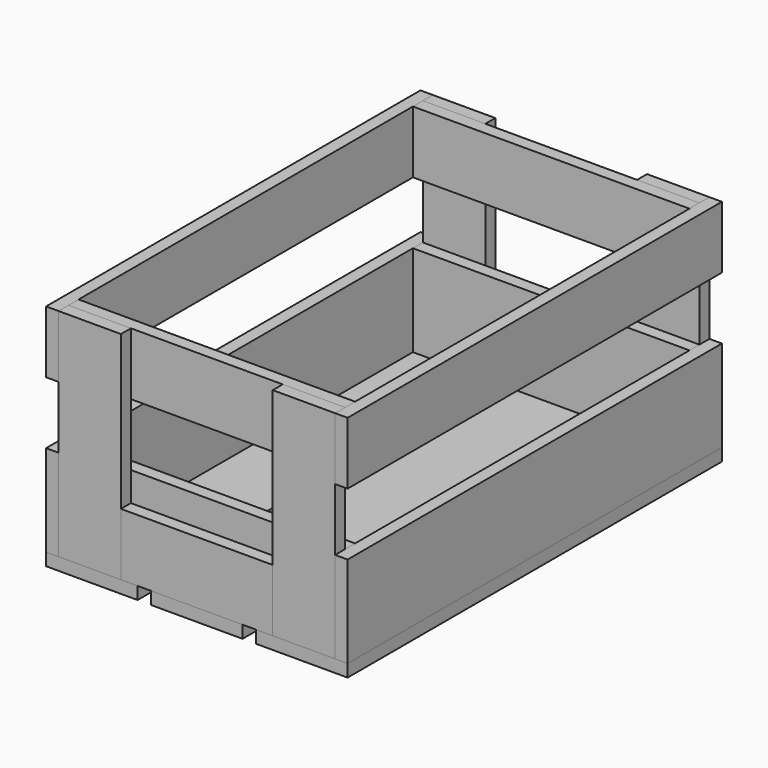
from build123d import *

# Parameters (mm, degrees)
F0_W      = 290
F0_H      = 225
F1_DEPTH  = 220
F2_W      = 12
F2_H      = 60
F3_DEPTH  = 450
F2_H_2    = 12
F2_W_2    = 88
F2_H_3    = 88
F4_DEPTH  = 450
F5_W      = 60
F5_H      = 12
F6_DEPTH  = 208
F5_W_2    = 73
F7_DEPTH  = 60
F8_START  = -120
F8_DEPTH  = 88
F9_DEPTH  = 12
F10_DEPTH = 25


with BuildPart() as f1:
    # F0 (on Top) → F1 (new body)
    with BuildSketch(Plane.XY):
        with Locations((145, 112.5)):
            Rectangle(F0_W, F0_H)
        with Locations((145, 337.5)):
            Rectangle(F0_W, F0_H)
    extrude(amount=F1_DEPTH)


with BuildPart() as f3:
    # F2 (on face) → F3 (new body, through all)
    with BuildSketch(Plane(origin=(0, 450, 0), x_dir=(-1, 0, 0), z_dir=(0, 1, 0))):
        with Locations((-284, 190)):
            Rectangle(F2_W, F2_H)
    extrude(amount=-F3_DEPTH)


with BuildPart() as f3b:
    # F2 (on face) → F3, piece 2 (new body, through all)
    with BuildSketch(Plane(origin=(0, 450, 0), x_dir=(-1, 0, 0), z_dir=(0, 1, 0))):
        Polygon((-278, 0), (-202, 0), (-202, 12), (-218, 12), (-278, 12), align=None)
        with Locations((-284, 6)):
            Rectangle(F2_W, F2_H_2)
    extrude(amount=-F3_DEPTH)


with BuildPart() as f3c:
    # F2 (on face) → F3, piece 3 (new body, through all)
    with BuildSketch(Plane(origin=(0, 450, 0), x_dir=(-1, 0, 0), z_dir=(0, 1, 0))):
        with Locations((-145, 6)):
            Rectangle(F2_W_2, F2_H_2)
    extrude(amount=-F3_DEPTH)


with BuildPart() as f3d:
    # F2 (on face) → F3, piece 4 (new body, through all)
    with BuildSketch(Plane(origin=(0, 450, 0), x_dir=(-1, 0, 0), z_dir=(0, 1, 0))):
        Polygon((-88, 0), (-12, 0), (-12, 12), (-72, 12), (-88, 12), align=None)
        with Locations((-6, 6)):
            Rectangle(F2_W, F2_H_2)
    extrude(amount=-F3_DEPTH)


with BuildPart() as f3e:
    # F2 (on face) → F3, piece 5 (new body, through all)
    with BuildSketch(Plane(origin=(0, 450, 0), x_dir=(-1, 0, 0), z_dir=(0, 1, 0))):
        with Locations((-6, 190)):
            Rectangle(F2_W, F2_H)
    extrude(amount=-F3_DEPTH)


with BuildPart() as f4:
    # F2 (on face) → F4 (new body, through all)
    with BuildSketch(Plane(origin=(0, 450, 0), x_dir=(-1, 0, 0), z_dir=(0, 1, 0))):
        with Locations((-284, 56)):
            Rectangle(F2_W, F2_H_3)
    extrude(amount=-F4_DEPTH)


with BuildPart() as f4b:
    # F2 (on face) → F4, piece 2 (new body, through all)
    with BuildSketch(Plane(origin=(0, 450, 0), x_dir=(-1, 0, 0), z_dir=(0, 1, 0))):
        with Locations((-6, 56)):
            Rectangle(F2_W, F2_H_3)
    extrude(amount=-F4_DEPTH)


with BuildPart() as f6:
    # F5 (on face) → F6 (new body, through all)
    with BuildSketch(Plane.XY.offset(220)):
        with Locations((42, 6)):
            Rectangle(F5_W, F5_H)
    extrude(amount=-F6_DEPTH)


with BuildPart() as f6b:
    # F5 (on face) → F6, piece 2 (new body, through all)
    with BuildSketch(Plane.XY.offset(220)):
        with Locations((248, 6)):
            Rectangle(F5_W, F5_H)
    extrude(amount=-F6_DEPTH)


with BuildPart() as f7:
    # F5 (on face) → F7 (new body)
    with BuildSketch(Plane.XY.offset(220)):
        with Locations((42, 18)):
            Rectangle(F5_W, F5_H)
        with Locations((108.5, 18)):
            Rectangle(F5_W_2, F5_H)
        with Locations((181.5, 18)):
            Rectangle(F5_W_2, F5_H)
        with Locations((248, 18)):
            Rectangle(F5_W, F5_H)
    extrude(amount=-F7_DEPTH)


with BuildPart() as f8:
    # F5 (on face) → F8 (new body)
    with BuildSketch(Plane.XY.offset(220).offset(F8_START)):
        with Locations((42, 18)):
            Rectangle(F5_W, F5_H)
        with Locations((108.5, 18)):
            Rectangle(F5_W_2, F5_H)
        with Locations((181.5, 18)):
            Rectangle(F5_W_2, F5_H)
        with Locations((248, 18)):
            Rectangle(F5_W, F5_H)
    extrude(amount=-F8_DEPTH)


with BuildPart() as f9:
    # F2 (on face) → F9 (new body)
    with BuildSketch(Plane(origin=(0, 450, 0), x_dir=(-1, 0, 0), z_dir=(0, 1, 0))):
        Polygon((-101, 12), (-88, 12), (-72, 12), (-72, 72), (-218, 72), (-218, 12), (-202, 12), (-189, 12), align=None)
    extrude(amount=-F9_DEPTH)


with BuildPart() as f10:
    # F0 (on Top) → F10 (new body)
    with BuildSketch(Plane.XY):
        with Locations((145, 112.5)):
            Rectangle(F0_W, F0_H)
    extrude(amount=F10_DEPTH)


with BuildPart() as f11_1:
    # F11: instance of F9
    add(f9.part.mirror(Plane(origin=(145, 225, 12.5), x_dir=(-1, 0, 0), z_dir=(0, 1, 0))))


with BuildPart() as f11_2:
    # F11: instance of F6b
    add(f6b.part.mirror(Plane(origin=(145, 225, 12.5), x_dir=(-1, 0, 0), z_dir=(0, 1, 0))))


with BuildPart() as f11_3:
    # F11: instance of F7
    add(f7.part.mirror(Plane(origin=(145, 225, 12.5), x_dir=(-1, 0, 0), z_dir=(0, 1, 0))))


with BuildPart() as f11_4:
    # F11: instance of F8
    add(f8.part.mirror(Plane(origin=(145, 225, 12.5), x_dir=(-1, 0, 0), z_dir=(0, 1, 0))))


with BuildPart() as f11_5:
    # F11: instance of F6
    add(f6.part.mirror(Plane(origin=(145, 225, 12.5), x_dir=(-1, 0, 0), z_dir=(0, 1, 0))))


solid = Compound([f3.part, f3b.part, f3c.part, f3d.part, f3e.part, f4.part, f4b.part, f6.part, f6b.part, f7.part, f8.part, f9.part, f11_1.part, f11_2.part, f11_3.part, f11_4.part, f11_5.part])
